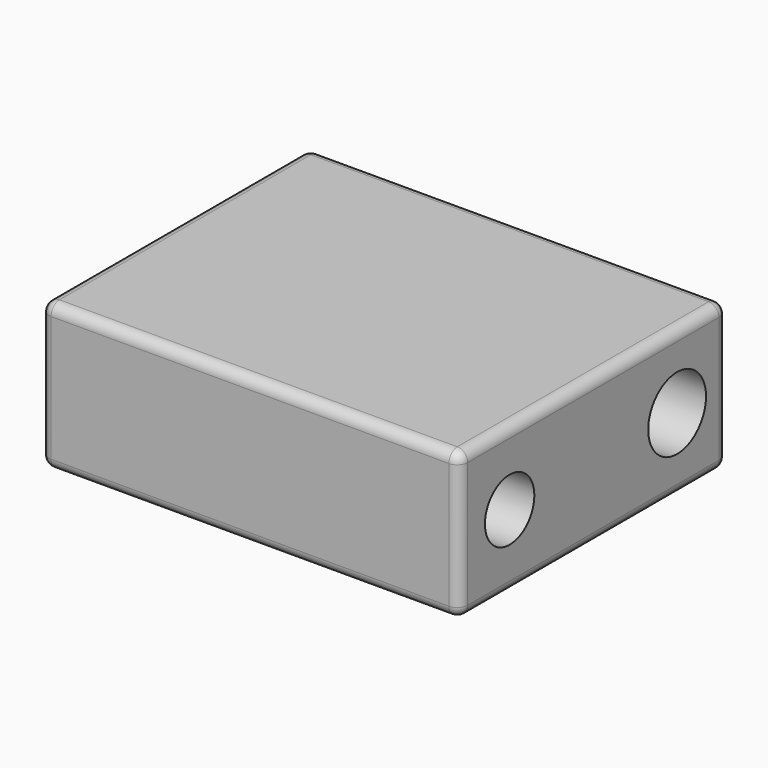
from build123d import *

# Parameters (mm, degrees)
F0_W         = 20
F0_H         = 16
F1_DEPTH     = 7
F2_R         = 0.5
F3_T1_DEPTH  = 22.5
F3_T3_DEPTH  = 16.75
F3_T5_DEPTH  = 6
F3_S9_W      = 0.5
F3_S9_H      = 0.5
F3_T10_DEPTH = 0.5
F3_S15_W     = 0.5
F3_S15_H     = 0.5
F3_T16_DEPTH = 0.5
F3_T20_ANGLE = 90
F3_T22_ANGLE = 90
F4_T1_DEPTH  = 6
F4_S5_W      = 0.5
F4_S5_H      = 0.5
F4_T6_DEPTH  = 0.5
F4_S11_W     = 0.5
F4_S11_H     = 0.5
F4_T12_DEPTH = 0.5
F5_T1_DEPTH  = 6
F5_S5_W      = 0.5
F5_S5_H      = 0.5
F5_T6_DEPTH  = 0.5
F5_S11_W     = 0.5
F5_S11_H     = 0.5
F5_T12_DEPTH = 0.5
F6_R         = 1.475
F6_R_2       = 1.725
F7_DEPTH     = 16.3


# Not quite as in the source:
# - a fillet or chamfer that OpenCascade refuses, or shapes differently, is made with other operations: its cross-section is extruded or revolved along the edge and cut away or added


with BuildPart() as f1:
    # F0 (on Top) → F1 (new body)
    with BuildSketch(Plane.XY):
        Rectangle(F0_W, F0_H)
    extrude(amount=-F1_DEPTH)

    # F2
    f2_edges = [f1.edges().sort_by_distance(p)[0] for p in [
        (0, 8, 0),
        (-10, 0, 0),
        (0, -8, 0),
        (10, 0, 0),
        (0, -8, -7),
    ]]
    fillet(f2_edges, radius=F2_R)

    # F3: fillet of radius 0.5 on 4 edges, made by hand

    # F3_s2 → F3_t1 (cut)
    with BuildSketch(Plane.YZ.offset(-11.25)):
        with BuildLine():
            ThreePointArc((8, -6.5), (7.8535533906, -6.8535533906), (7.5, -7))
            Line((7.5, -7), (8, -7))
            Line((8, -7), (8, -6.5))
        make_face()
    extrude(amount=F3_T1_DEPTH, mode=Mode.SUBTRACT)

    # F3_s4 → F3_t3 (cut)
    with BuildSketch(Plane.XZ.offset(-9.25)):
        with BuildLine():
            ThreePointArc((-9.5, -7), (-9.8535533906, -6.8535533906), (-10, -6.5))
            Line((-10, -6.5), (-10, -7))
            Line((-10, -7), (-9.5, -7))
        make_face()
        with BuildLine():
            ThreePointArc((10, -6.5), (9.8535533906, -6.8535533906), (9.5, -7))
            Line((9.5, -7), (10, -7))
            Line((10, -7), (10, -6.5))
        make_face()
    extrude(amount=F3_T3_DEPTH, mode=Mode.SUBTRACT)

    # F3_s6 → F3_t5 (cut)
    with BuildSketch(Plane.XY.offset(-6.5)):
        with BuildLine():
            ThreePointArc((10, -7.5), (9.8535533906, -7.8535533906), (9.5, -8))
            Line((9.5, -8), (10, -8))
            Line((10, -8), (10, -7.5))
        make_face()
        with BuildLine():
            ThreePointArc((-10, -7.5), (-9.8535533906, -7.8535533906), (-9.5, -8))
            Line((-9.5, -8), (-10, -8))
            Line((-10, -8), (-10, -7.5))
        make_face()
    extrude(amount=F3_T5_DEPTH, mode=Mode.SUBTRACT)


with BuildPart() as f3_tool8:
    # F3_s9 → F3_t10 (new body)
    with BuildSketch(Plane.YZ.offset(9.5)):
        with Locations((-7.75, -0.25)):
            Rectangle(F3_S9_W, F3_S9_H)
    extrude(amount=F3_T10_DEPTH)

    # F3_s11 → F3_t12 (revolve, cut)
    with BuildSketch(Plane(origin=(9.5, -7.5, -0.5), x_dir=(0, 0.7071067812, -0.7071067812), z_dir=(0, -0.7071067812, -0.7071067812))):
        with BuildLine():
            ThreePointArc((0, -0.5), (0.5, 0), (0, 0.5))
            Line((0, 0.5), (0, -0.5))
        make_face()
    revolve(axis=Axis((9.5, -7.5, -0.5), (1, 0, 0)), mode=Mode.SUBTRACT)


with BuildPart() as f1_1:
    add(f1.part)

    # F3_t7: cut F3_tool8
    add(f3_tool8.part, mode=Mode.SUBTRACT)


with BuildPart() as f3_tool14:
    # F3_s15 → F3_t16 (new body)
    with BuildSketch(Plane.YZ.offset(-9.5)):
        with Locations((-7.75, -0.25)):
            Rectangle(F3_S15_W, F3_S15_H)
    extrude(amount=-F3_T16_DEPTH)

    # F3_s17 → F3_t18 (revolve, cut)
    with BuildSketch(Plane(origin=(-9.5, -7.5, -0.5), x_dir=(0, 0.7071067812, -0.7071067812), z_dir=(0, 0.7071067812, 0.7071067812))):
        with BuildLine():
            ThreePointArc((0, -0.5), (0.5, 0), (0, 0.5))
            Line((0, 0.5), (0, -0.5))
        make_face()
    revolve(axis=Axis((-9.5, -7.5, -0.5), (-1, 0, 0)), mode=Mode.SUBTRACT)


with BuildPart() as f1_2:
    add(f1_1.part)

    # F3_t13: cut F3_tool14
    add(f3_tool14.part, mode=Mode.SUBTRACT)

    # F3_s19 → F3_t20 (revolve, cut)
    with BuildSketch(Plane.XY.offset(-6.5)):
        with BuildLine():
            ThreePointArc((10, -7.5), (9.8535533906, -7.8535533906), (9.5, -8))
            Line((9.5, -8), (10, -8))
            Line((10, -8), (10, -7.5))
        make_face()
    revolve(axis=Axis((10, -7.5, -6.5), (1, 0, 0)), revolution_arc=F3_T20_ANGLE, mode=Mode.SUBTRACT)

    # F3_s21 → F3_t22 (revolve, cut)
    with BuildSketch(Plane.XY.offset(-6.5)):
        with BuildLine():
            ThreePointArc((-10, -7.5), (-9.8535533906, -7.8535533906), (-9.5, -8))
            Line((-9.5, -8), (-10, -8))
            Line((-10, -8), (-10, -7.5))
        make_face()
    revolve(axis=Axis((-10, -7.5, -6.5), (1, 0, 0)), revolution_arc=F3_T22_ANGLE, mode=Mode.SUBTRACT)

    # F4: fillet of radius 0.5 on 1 edges, made by hand

    # F4_s2 → F4_t1 (cut)
    with BuildSketch(Plane.XY.offset(-6.5)):
        with BuildLine():
            ThreePointArc((-9.5, 8), (-9.8535533906, 7.8535533906), (-10, 7.5))
            Line((-10, 7.5), (-10, 8))
            Line((-10, 8), (-9.5, 8))
        make_face()
    extrude(amount=F4_T1_DEPTH, mode=Mode.SUBTRACT)


with BuildPart() as f4_tool4:
    # F4_s5 → F4_t6 (new body)
    with BuildSketch(Plane.XZ.offset(-7.5)):
        with Locations((-9.75, -0.25)):
            Rectangle(F4_S5_W, F4_S5_H)
    extrude(amount=-F4_T6_DEPTH)

    # F4_s7 → F4_t8 (revolve, cut)
    with BuildSketch(Plane(origin=(-9.5, 7.5, -0.5), x_dir=(0.7071067812, 0, -0.7071067812), z_dir=(0.7071067812, 0, 0.7071067812))):
        with BuildLine():
            ThreePointArc((0, -0.5), (0.5, 0), (0, 0.5))
            Line((0, 0.5), (0, -0.5))
        make_face()
    revolve(axis=Axis((-9.5, 7.5, -0.5), (0, 1, 0)), mode=Mode.SUBTRACT)


with BuildPart() as f1_3:
    add(f1_2.part)

    # F4_t3: cut F4_tool4
    add(f4_tool4.part, mode=Mode.SUBTRACT)


with BuildPart() as f4_tool10:
    # F4_s11 → F4_t12 (new body)
    with BuildSketch(Plane.XZ.offset(-7.5)):
        with Locations((-9.75, -6.75)):
            Rectangle(F4_S11_W, F4_S11_H)
    extrude(amount=-F4_T12_DEPTH)

    # F4_s13 → F4_t14 (revolve, cut)
    with BuildSketch(Plane(origin=(-9.5, 7.5, -6.5), x_dir=(0.7071067812, 0, 0.7071067812), z_dir=(-0.7071067812, 0, 0.7071067812))):
        with BuildLine():
            ThreePointArc((0, -0.5), (0.5, 0), (0, 0.5))
            Line((0, 0.5), (0, -0.5))
        make_face()
    revolve(axis=Axis((-9.5, 7.5, -6.5), (0, 1, 0)), mode=Mode.SUBTRACT)


with BuildPart() as f1_4:
    add(f1_3.part)

    # F4_t9: cut F4_tool10
    add(f4_tool10.part, mode=Mode.SUBTRACT)

    # F5: fillet of radius 0.5 on 1 edges, made by hand

    # F5_s2 → F5_t1 (cut)
    with BuildSketch(Plane.XY.offset(-6.5)):
        with BuildLine():
            ThreePointArc((9.5, 8), (9.8535533906, 7.8535533906), (10, 7.5))
            Line((10, 7.5), (10, 8))
            Line((10, 8), (9.5, 8))
        make_face()
    extrude(amount=F5_T1_DEPTH, mode=Mode.SUBTRACT)


with BuildPart() as f5_tool4:
    # F5_s5 → F5_t6 (new body)
    with BuildSketch(Plane.XZ.offset(-7.5)):
        with Locations((9.75, -0.25)):
            Rectangle(F5_S5_W, F5_S5_H)
    extrude(amount=-F5_T6_DEPTH)

    # F5_s7 → F5_t8 (revolve, cut)
    with BuildSketch(Plane(origin=(9.5, 7.5, -0.5), x_dir=(-0.7071067812, 0, -0.7071067812), z_dir=(0.7071067812, 0, -0.7071067812))):
        with BuildLine():
            ThreePointArc((0, -0.5), (0.5, 0), (0, 0.5))
            Line((0, 0.5), (0, -0.5))
        make_face()
    revolve(axis=Axis((9.5, 7.5, -0.5), (0, 1, 0)), mode=Mode.SUBTRACT)


with BuildPart() as f1_5:
    add(f1_4.part)

    # F5_t3: cut F5_tool4
    add(f5_tool4.part, mode=Mode.SUBTRACT)


with BuildPart() as f5_tool10:
    # F5_s11 → F5_t12 (new body)
    with BuildSketch(Plane.XZ.offset(-7.5)):
        with Locations((9.75, -6.75)):
            Rectangle(F5_S11_W, F5_S11_H)
    extrude(amount=-F5_T12_DEPTH)

    # F5_s13 → F5_t14 (revolve, cut)
    with BuildSketch(Plane(origin=(9.5, 7.5, -6.5), x_dir=(-0.7071067812, 0, 0.7071067812), z_dir=(-0.7071067812, 0, -0.7071067812))):
        with BuildLine():
            ThreePointArc((0, -0.5), (0.5, 0), (0, 0.5))
            Line((0, 0.5), (0, -0.5))
        make_face()
    revolve(axis=Axis((9.5, 7.5, -6.5), (0, 1, 0)), mode=Mode.SUBTRACT)


with BuildPart() as f1_6:
    add(f1_5.part)

    # F5_t9: cut F5_tool10
    add(f5_tool10.part, mode=Mode.SUBTRACT)

    # F6 (on face) → F7 (cut)
    with BuildSketch(Plane.YZ.offset(10)):
        with Locations((-5, -3.5)):
            Circle(F6_R)
        with Locations((5, -3.5)):
            Circle(F6_R_2)
    extrude(amount=-F7_DEPTH, mode=Mode.SUBTRACT)


solid = f1_6.part
